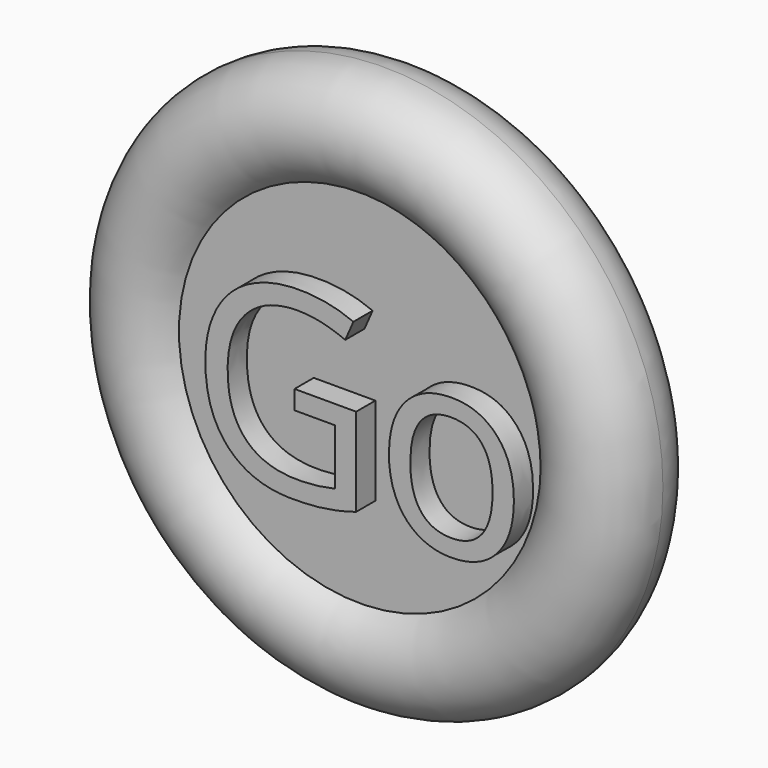
from build123d import *

# Parameters (mm, degrees)
F2_TEXT_SIZE = 46.4743611196
F3_DEPTH     = 5
F4_TEXT_SIZE = 52.8846194761
F5_DEPTH     = 5


# Not quite as in the source:
# - Text() gives the source's letters only with a copy of the font that has no kerning and outlines rounded to 1/6400 em; it was checked with that copy


with BuildPart() as f1:
    # F0 (on Top) → F1 (revolve)
    with BuildSketch(Plane.XY):
        with BuildLine():
            Line((-4.7435319049, 35.7692316175), (-42.4038507044, 35.7692316175))
            Line((-42.4038507044, 35.7692316175), (-42.4038507044, 23.2692323625))
            Line((-42.4038507044, 23.2692323625), (-4.7435319049, 23.2692323625))
            ThreePointArc((-4.7435319049, 23.2692323625), (-6.6549029537, 29.51923199), (-4.7435319049, 35.7692316175))
        make_face()
        with BuildLine():
            Line((12.9807703197, 35.7692316175), (-4.7435319049, 35.7692316175))
            ThreePointArc((-4.7435319049, 35.7692316175), (-6.6549029537, 29.51923199), (-4.7435319049, 23.2692323625))
            Line((-4.7435319049, 23.2692323625), (12.9807703197, 23.2692323625))
            Line((12.9807703197, 23.2692323625), (12.9807703197, 35.7692316175))
        make_face()
        with BuildLine():
            ThreePointArc((15.6933661886, 29.51923199), (7.7870992184, 40.20484497), (-4.7435319049, 35.7692316175))
            Line((-4.7435319049, 35.7692316175), (12.9807703197, 35.7692316175))
            Line((12.9807703197, 35.7692316175), (12.9807703197, 23.2692323625))
            Line((12.9807703197, 23.2692323625), (-4.7435319049, 23.2692323625))
            ThreePointArc((-4.7435319049, 23.2692323625), (7.7870992184, 18.83361901), (15.6933661886, 29.51923199))
        make_face()
    revolve(axis=Axis((-42.4038507044, 29.51923199, 0), (0, -1, 0)))

    # F2 (on face) → F3 (join)
    with BuildSketch(Plane(origin=(0, 35.7692316175, 0), x_dir=(-1, 0, 0), z_dir=(0, 1, 0))):
        with Locations((-5.2917618304, -15.0579875335)):
            Text('stop', F2_TEXT_SIZE, font='Open Sans', text_align=(TextAlign.LEFT, TextAlign.BOTTOM))
    extrude(amount=F3_DEPTH)

    # F4 (on face) → F5 (join)
    with BuildSketch(Plane.XZ.offset(-23.2692323625)):
        with Locations((-73.8082281314, -19.2307699472)):
            Text('Go', F4_TEXT_SIZE, font='Open Sans', text_align=(TextAlign.LEFT, TextAlign.BOTTOM))
    extrude(amount=F5_DEPTH)


solid = f1.part
